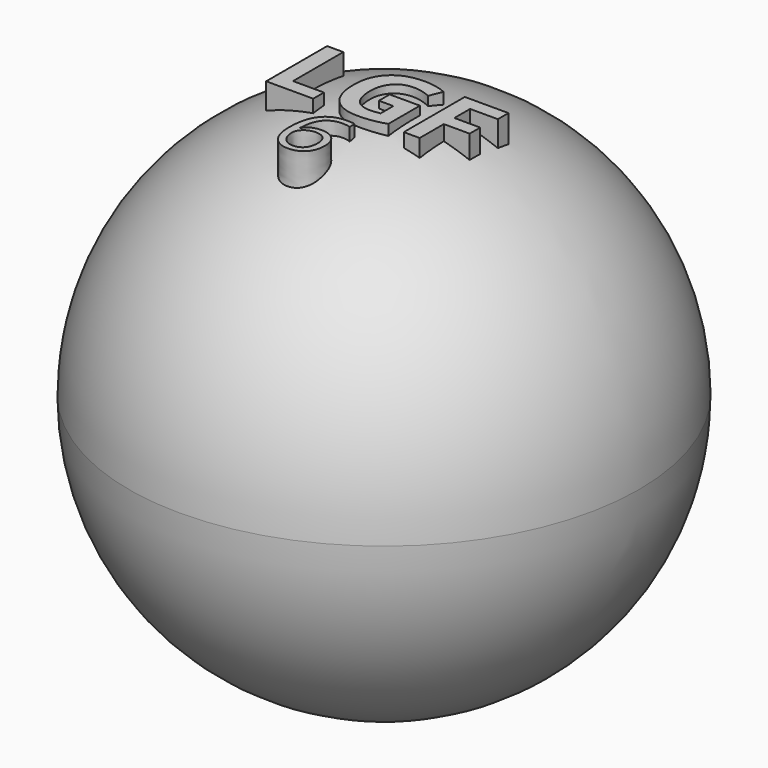
from build123d import *

# Parameters (mm, degrees)
F2_TEXT_SIZE   = 23.9275350598
F2_TEXT_SIZE_2 = 20.0163029755
F3_DEPTH       = 25.4
F4_DEPTH       = 58.674


# Not quite as in the source:
# - Text() gives the source's letters only with a copy of the font that has no kerning and outlines rounded to 1/6400 em; it was checked with that copy


with BuildPart() as f1:
    # F0 (on Front) → F1 (revolve)
    with BuildSketch(Plane.XZ):
        with BuildLine():
            ThreePointArc((0, -57.15), (40.4111525448, -40.4111525448), (57.15, 0))
            ThreePointArc((57.15, 0), (40.4111525448, 40.4111525448), (0, 57.15))
            Line((0, 57.15), (0, -57.15))
        make_face()
    revolve(axis=Axis((0, 0, 0), (0, 0, -1)))



with BuildPart() as f3:
    # F2 (on Top) → F3 (new body)
    with BuildSketch(Plane.XY):
        with Locations((-22.1973915905, -7.951303036)):
            Text('LGF', F2_TEXT_SIZE, font='Open Sans', font_style=FontStyle.BOLD, text_align=(TextAlign.LEFT, TextAlign.BOTTOM))
        with Locations((-7.2000294915, -25.2314712852)):
            Text('6', F2_TEXT_SIZE_2, font='Open Sans', text_align=(TextAlign.LEFT, TextAlign.BOTTOM))
    extrude(amount=F3_DEPTH)


with BuildPart() as f1_1:
    add(f1.part)

    add(f3.part)  # F4 merges F3
    # F2 (on Top) → F4 (join)
    with BuildSketch(Plane.XY):
        with Locations((-22.1973915905, -7.951303036)):
            Text('LGF', F2_TEXT_SIZE, font='Open Sans', font_style=FontStyle.BOLD, text_align=(TextAlign.LEFT, TextAlign.BOTTOM))
        with Locations((-7.2000294915, -25.2314712852)):
            Text('6', F2_TEXT_SIZE_2, font='Open Sans', text_align=(TextAlign.LEFT, TextAlign.BOTTOM))
    extrude(amount=F4_DEPTH)


solid = f1_1.part
